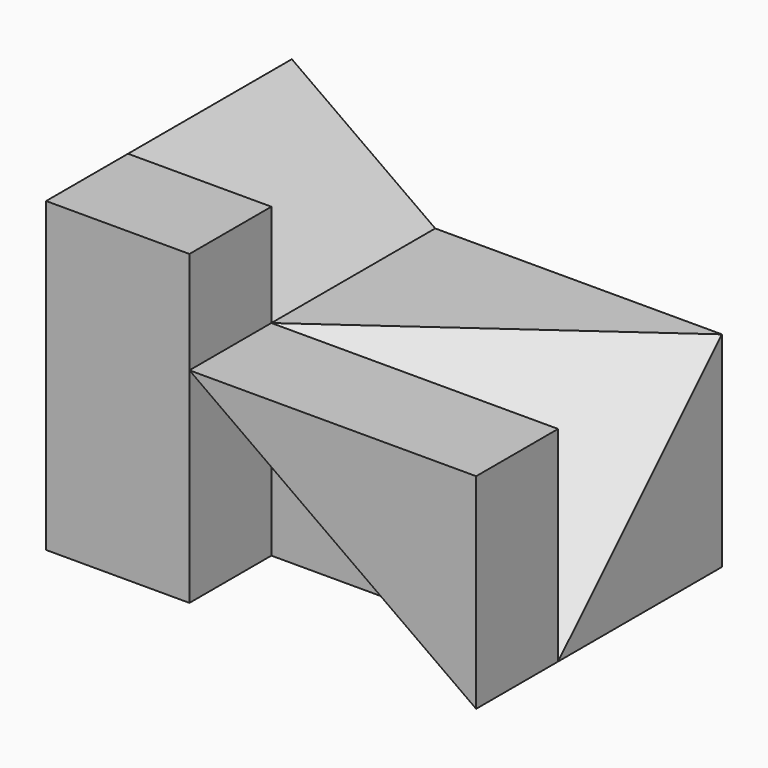
from build123d import *

# Parameters (mm, degrees)
F1_DEPTH  = 30
F3_DEPTH  = 20
F5_DEPTH  = 10
F8_DEPTH  = 25.2477497707
F9_DEPTH  = 10
F10_DEPTH = 10


with BuildPart() as f1:
    # F0 (on Front) → F1 (new body)
    with BuildSketch(Plane.XZ):
        Polygon((0, 30), (0, 0), (42, 0), (42, 20), (14, 20), (14, 30), align=None)
    extrude(amount=F1_DEPTH)

    # F2 (on face) → F3 (cut)
    with BuildSketch(Plane(origin=(0, 0, 0), x_dir=(-1, 0, 0), z_dir=(0, 1, 0))):
        Polygon((-14, 20), (0, 30), (-14, 30), align=None)
    extrude(amount=-F3_DEPTH, mode=Mode.SUBTRACT)

    # F4 (on face) → F5 (cut)
    with BuildSketch(Plane.XZ.offset(30)):
        Polygon((42, 20), (14, 20), (42, 0), align=None)
    extrude(amount=-F5_DEPTH, mode=Mode.SUBTRACT)

    # F7 (on 3pt) → F8 (cut, through all)
    with BuildSketch(Plane(origin=(14.2276422764, -19.918699187, 19.918699187), x_dir=(0.8926073983, 0.3187883565, -0.3187883565), z_dir=(0.4508348173, -0.6311687443, 0.6311687443))):
        Polygon((31.1137435975, 14.1421356237), (-0.2550306852, 0), (31.1137435975, -14.1421356237), align=None)
    extrude(amount=F8_DEPTH, mode=Mode.SUBTRACT)

    # F4 (on face) → F9 (join, through all)
    with BuildSketch(Plane.XZ.offset(30)):
        Polygon((42, 20), (14, 20), (42, 0), align=None)
    extrude(amount=-F9_DEPTH)

    # F4 (on face) → F10 (cut, through all)
    with BuildSketch(Plane.XZ.offset(30)):
        Polygon((42, 0), (14, 20), (14, 0), align=None)
    extrude(amount=-F10_DEPTH, mode=Mode.SUBTRACT)


solid = f1.part
